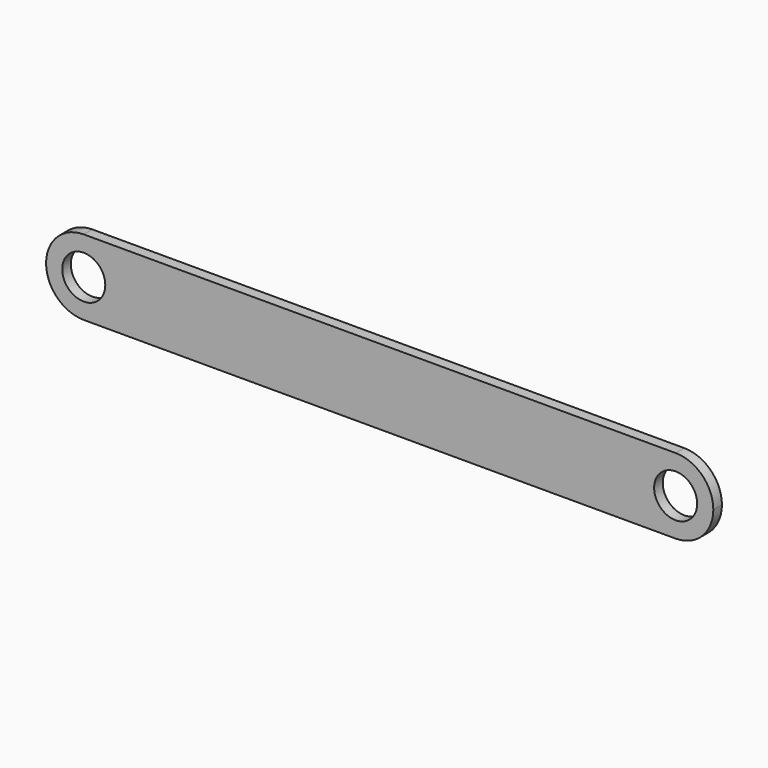
from build123d import *

# Parameters (mm, degrees)
F0_W     = 124
F0_H     = 14
F1_DEPTH = 2
F2_R     = 4
F3_DEPTH = 25
F4_R     = 4
F5_DEPTH = 25
F6_R     = 6.99999


# Not quite as in the source:
# - a fillet or chamfer is up to 0.001 mm smaller than in the source, because OpenCascade refuses the exact size


with BuildPart() as f1:
    # F0 (on Front) → F1 (new body)
    with BuildSketch(Plane.XZ):
        Rectangle(F0_W, F0_H)
    extrude(amount=F1_DEPTH)

    # F2 (on face) → F3 (cut)
    with BuildSketch(Plane.XZ.offset(2)):
        with Locations((-55, 0)):
            Circle(F2_R)
    extrude(amount=-F3_DEPTH, mode=Mode.SUBTRACT)

    # F4 (on face) → F5 (cut)
    with BuildSketch(Plane.XZ.offset(2)):
        with Locations((55, 0)):
            Circle(F4_R)
    extrude(amount=-F5_DEPTH, mode=Mode.SUBTRACT)

    # F6 (radius 7 in the source; OpenCascade refuses exactly that, so slightly less here)
    f6_edges = [f1.edges().sort_by_distance(p)[0] for p in [
        (-62, -1, 7),
        (-62, -1, -7),
        (62, -1, 7),
        (62, -1, -7),
    ]]
    fillet(f6_edges, radius=F6_R)


solid = f1.part
